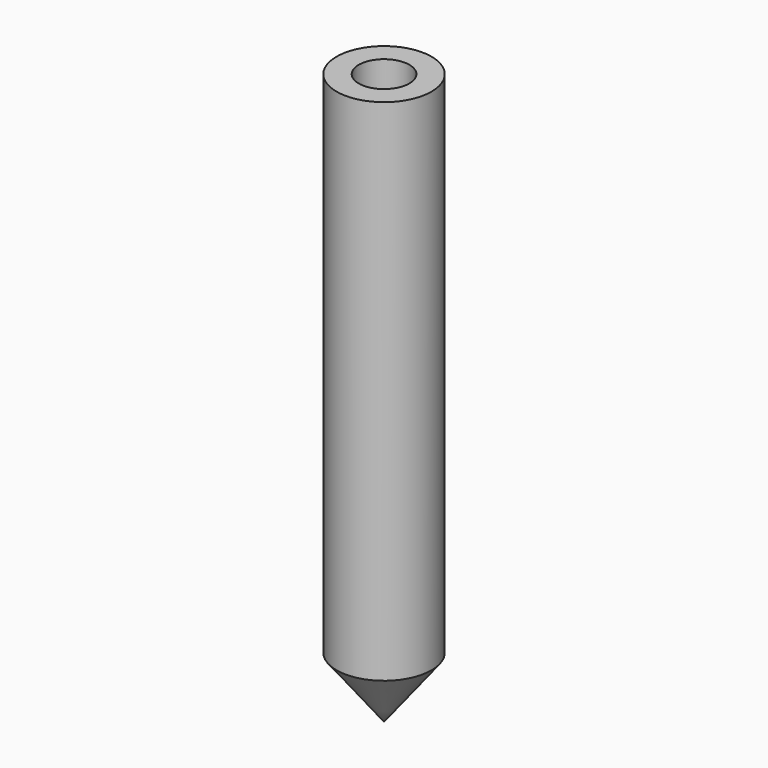
from build123d import *

# Parameters (mm, degrees)
F0_R     = 6
F0_R_2   = 3.2
F1_DEPTH = 64.4
F2_R     = 5.25
F2_R_2   = 4
F3_DEPTH = 63
F4_R     = 6
F4_R_2   = 5.25
F4_R_3   = 3.2
F5_DEPTH = 7.7
F6_R     = 3.2
F7_DEPTH = 7.7


# Not quite as in the source:
# - a fillet or chamfer that OpenCascade refuses, or shapes differently, is made with other operations: its cross-section is extruded or revolved along the edge and cut away or added


with BuildPart() as f1:
    # F0 (on Top) → F1 (new body)
    with BuildSketch(Plane.XY):
        Circle(F0_R)
        Circle(F0_R_2, mode=Mode.SUBTRACT)
    extrude(amount=-F1_DEPTH)

    # F2 (on face) → F3 (cut)
    with BuildSketch(Plane(origin=(0, 0, -64.4), x_dir=(1, 0, 0), z_dir=(0, 0, -1))):
        Circle(F2_R)
        Circle(F2_R_2, mode=Mode.SUBTRACT)
    extrude(amount=-F3_DEPTH, mode=Mode.SUBTRACT)


with BuildPart() as f5:
    # F4 (on face) → F5 (new body)
    with BuildSketch(Plane(origin=(0, 0, -64.4), x_dir=(1, 0, 0), z_dir=(0, 0, -1))):
        Circle(F4_R)
        Circle(F4_R_2, mode=Mode.SUBTRACT)
        Circle(F4_R_2)
        Circle(F4_R_3, mode=Mode.SUBTRACT)
    extrude(amount=F5_DEPTH)

    # F6 (on face) → F7 (join)
    with BuildSketch(Plane(origin=(0, 0, -72.1), x_dir=(1, 0, 0), z_dir=(0, 0, -1))):
        Circle(F6_R)
    extrude(amount=-F7_DEPTH)

    # F8: chamfer of 7.7 x 6 on 1 edges, made by hand

    # F8_s1 → F8_t2 (revolve, cut)
    with BuildSketch(Plane.XZ):
        Polygon((6, -64.4), (0, -72.1), (6, -72.1), align=None)
    revolve(axis=Axis((0, 0, -72.1), (0, 0, -1)), mode=Mode.SUBTRACT)


solid = Compound([f1.part, f5.part])
